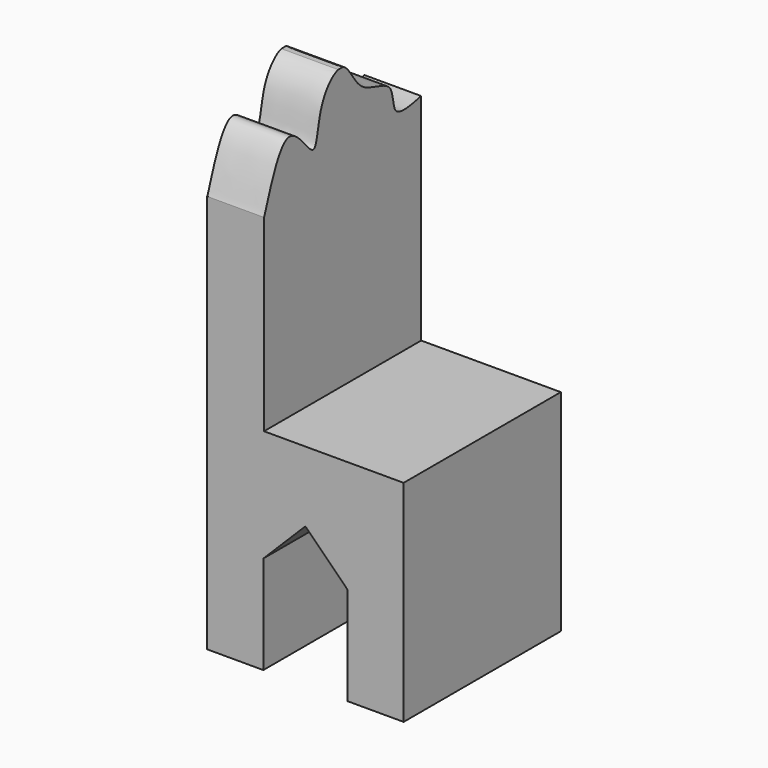
from build123d import *

# Parameters (mm, degrees)
F1_W        = 14
F1_H        = 14
F2_DEPTH    = 15
F3_W        = 4.0493770838
F3_H        = 14
F4_DEPTH    = 20
F6_DEPTH    = 25
F7_W        = 5.9968179464
F7_H        = 10
F8_DEPTH    = 25
F9_T1_DEPTH = 14


# Not quite as in the source:
# - a fillet or chamfer that OpenCascade refuses, or shapes differently, is made with other operations: its cross-section is extruded or revolved along the edge and cut away or added


with BuildPart() as f2:
    # F1 (on offset) → F2 (new body)
    with BuildSketch(Plane.XY.offset(6)):
        with Locations((-104.1826612949, -17.1571627557)):
            Rectangle(F1_W, F1_H)
    extrude(amount=F2_DEPTH)

    # F3 (on face) → F4 (join)
    with BuildSketch(Plane.XY.offset(21)):
        with Locations((-109.157972753, -17.1571627557)):
            Rectangle(F3_W, F3_H)
    extrude(amount=F4_DEPTH)

    # F5 (on face) → F6 (cut)
    with BuildSketch(Plane(origin=(-111.1826612949, 0, 0), x_dir=(0, -1, 0), z_dir=(-1, 0, 0))):
        with BuildLine():
            Line((10.1571627557, 41), (10.1571627557, 36.341752857))
            add(Edge.make_bspline(
                [(10.1571627557, 36.341752857), (11.1036728702, 36.1359380459), (12.8808040357, 35.7495080338), (12.4312722311, 38.5838720764), (15.8432736879, 38.466470991), (16.5506011139, 40.811261571), (17.1571627557, 41)],
                knots=[0, 0, 0, 0, 0.1074764373, 0.2017936453, 0.3194916252, 0.4343555632, 0.4343555632, 0.4343555632, 0.4343555632], degree=3))
            Line((17.1571627557, 41), (10.1571627557, 41))
        make_face()
        with BuildLine():
            add(Edge.make_bspline(
                [(17.1571627557, 41), (17.2807406542, 41.0384526432), (17.4149947295, 41.0366686909), (17.5538311602, 41)],
                knots=[0.4343555632, 0.4343555632, 0.4343555632, 0.4343555632, 0.4577573794, 0.4577573794, 0.4577573794, 0.4577573794], degree=3))
            Line((17.1571627557, 41), (17.5538311602, 41))
        make_face()
        with BuildLine():
            Line((24.1571627557, 41), (17.5538311602, 41))
            add(Edge.make_bspline(
                [(17.5538311602, 41), (18.0819152443, 40.860525426), (19.4476463077, 39.3803759727), (19.3611823544, 35.2887382601), (22.4135127849, 41.0203121515), (23.9648709709, 34.6951006825), (24.1571627557, 34.419786185)],
                knots=[0.4577573794, 0.4577573794, 0.4577573794, 0.4577573794, 0.5467695113, 0.6622841032, 0.7808817799, 0.9350414154, 0.9350414154, 0.9350414154, 0.9350414154], degree=3))
            Line((24.1571627557, 34.419786185), (24.1571627557, 35.2434851229))
            Line((24.1571627557, 35.2434851229), (24.1571627557, 41))
        make_face()
    extrude(amount=-F6_DEPTH, mode=Mode.SUBTRACT)

    # F7 (on face) → F8 (cut)
    with BuildSketch(Plane.XZ.offset(24.1571627557)):
        with Locations((-104.1842523217, 11)):
            Rectangle(F7_W, F7_H)
    extrude(amount=-F8_DEPTH, mode=Mode.SUBTRACT)

    # F9: chamfer of 3 on 2 edges, made by hand

    # F9_s2 → F9_t1 (join)
    with BuildSketch(Plane.XZ.offset(10.1571627557)):
        with BuildLine():
            Line((-104.0978084812, 16.0848528137), (-107.2675141087, 12.9151471863))
            Line((-107.2675141087, 12.9151471863), (-107.3275141087, 12.9151471863))
            ThreePointArc((-107.3275141087, 12.9151471863), (-107.2426612949, 14.4575735931), (-107.2426612949, 16))
            Line((-107.2426612949, 16), (-107.1826612949, 16.06))
            ThreePointArc((-107.1826612949, 16.06), (-105.6402348881, 16.06), (-104.0978084812, 16.1448528137))
            Line((-104.0978084812, 16.1448528137), (-104.0978084812, 16.0848528137))
        make_face()
        with BuildLine():
            Line((-101.1009905348, 12.9151471863), (-104.2706961622, 16.0848528137))
            Line((-104.2706961622, 16.0848528137), (-104.2706961622, 16.1448528137))
            ThreePointArc((-104.2706961622, 16.1448528137), (-102.7282697554, 16.06), (-101.1858433485, 16.06))
            Line((-101.1858433485, 16.06), (-101.1258433485, 16))
            ThreePointArc((-101.1258433485, 16), (-101.1258433485, 14.4575735931), (-101.0409905348, 12.9151471863))
            Line((-101.0409905348, 12.9151471863), (-101.1009905348, 12.9151471863))
        make_face()
    extrude(amount=F9_T1_DEPTH)


solid = f2.part
